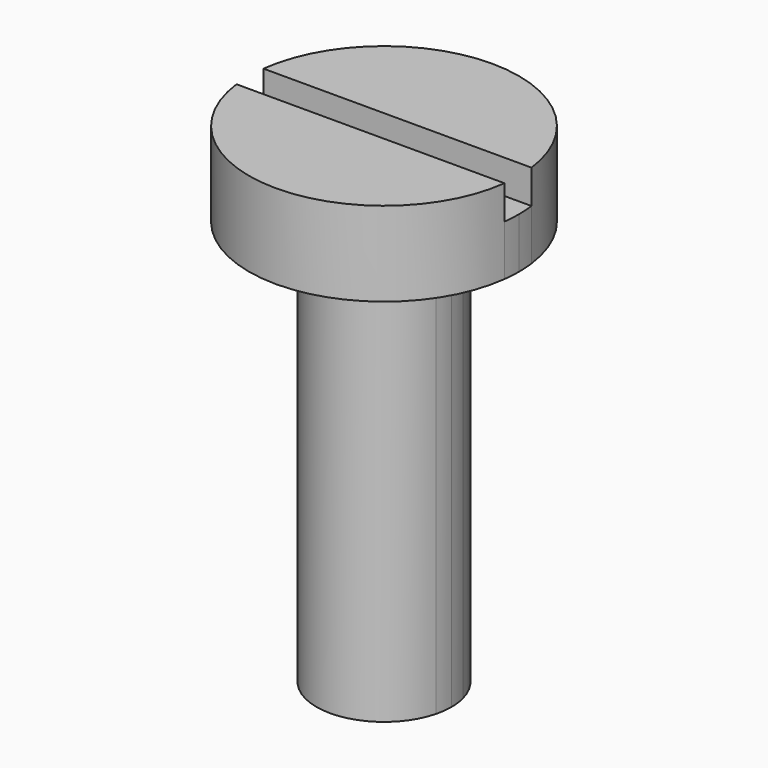
from build123d import *

# Parameters (mm, degrees)
F1_DEPTH = 12
F2_DEPTH = 2.5
F3_DEPTH = 1.5


# Not quite as in the source:
# - a feature names something its author has since deleted; it is built from what else it names


with BuildPart() as f1:
    # F0 (on Top) → F1 (new body)
    with BuildSketch(Plane.XY):
        with BuildLine():
            Line((-1.9364916731, 0.5), (1.9364916731, 0.5))
            ThreePointArc((1.9364916731, 0.5), (0, 2), (-1.9364916731, 0.5))
        make_face()
        with BuildLine():
            ThreePointArc((2, 0), (1.9840593925, 0.252008585), (1.9364916731, 0.5))
            Line((1.9364916731, 0.5), (-1.9364916731, 0.5))
            ThreePointArc((-1.9364916731, 0.5), (-2, 0), (-1.9364916731, -0.5))
            Line((-1.9364916731, -0.5), (1.9364916731, -0.5))
            ThreePointArc((1.9364916731, -0.5), (1.9840593925, -0.252008585), (2, 0))
        make_face()
        with BuildLine():
            ThreePointArc((-1.9364916731, -0.5), (0, -2), (1.9364916731, -0.5))
            Line((1.9364916731, -0.5), (-1.9364916731, -0.5))
        make_face()
    extrude(amount=-F1_DEPTH)

    # F0 (on Top) → F2 (join)
    with BuildSketch(Plane.XY):
        with BuildLine():
            ThreePointArc((-3.9686269666, -0.5), (0, -4), (3.9686269666, -0.5))
            Line((3.9686269666, -0.5), (1.9364916731, -0.5))
            ThreePointArc((1.9364916731, -0.5), (0, -2), (-1.9364916731, -0.5))
            Line((-1.9364916731, -0.5), (-3.9686269666, -0.5))
        make_face()
        with BuildLine():
            Line((1.9364916731, 0.5), (3.9686269666, 0.5))
            ThreePointArc((3.9686269666, 0.5), (0, 4), (-3.9686269666, 0.5))
            Line((-3.9686269666, 0.5), (-1.9364916731, 0.5))
            ThreePointArc((-1.9364916731, 0.5), (0, 2), (1.9364916731, 0.5))
        make_face()
        with BuildLine():
            Line((-1.9364916731, 0.5), (1.9364916731, 0.5))
            ThreePointArc((1.9364916731, 0.5), (0, 2), (-1.9364916731, 0.5))
        make_face()
        with BuildLine():
            ThreePointArc((-1.9364916731, -0.5), (0, -2), (1.9364916731, -0.5))
            Line((1.9364916731, -0.5), (-1.9364916731, -0.5))
        make_face()
    extrude(amount=F2_DEPTH)

    # F0 (on Top) → F3 (join)
    with BuildSketch(Plane.XY):
        with BuildLine():
            Line((-1.9364916731, 0.5), (-3.9686269666, 0.5))
            ThreePointArc((-3.9686269666, 0.5), (-4, 0), (-3.9686269666, -0.5))
            Line((-3.9686269666, -0.5), (-1.9364916731, -0.5))
            ThreePointArc((-1.9364916731, -0.5), (-2, 0), (-1.9364916731, 0.5))
        make_face()
        with BuildLine():
            ThreePointArc((2, 0), (1.9840593925, 0.252008585), (1.9364916731, 0.5))
            Line((1.9364916731, 0.5), (-1.9364916731, 0.5))
            ThreePointArc((-1.9364916731, 0.5), (-2, 0), (-1.9364916731, -0.5))
            Line((-1.9364916731, -0.5), (1.9364916731, -0.5))
            ThreePointArc((1.9364916731, -0.5), (1.9840593925, -0.252008585), (2, 0))
        make_face()
        with BuildLine():
            ThreePointArc((3.9686269666, -0.5), (3.9921490369, -0.2504916502), (4, 0))
            ThreePointArc((4, 0), (3.9921490369, 0.2504916502), (3.9686269666, 0.5))
            Line((3.9686269666, 0.5), (1.9364916731, 0.5))
            ThreePointArc((1.9364916731, 0.5), (1.9840593925, 0.252008585), (2, 0))
            ThreePointArc((2, 0), (1.9840593925, -0.252008585), (1.9364916731, -0.5))
            Line((1.9364916731, -0.5), (3.9686269666, -0.5))
        make_face()
    extrude(amount=F3_DEPTH)


solid = f1.part
